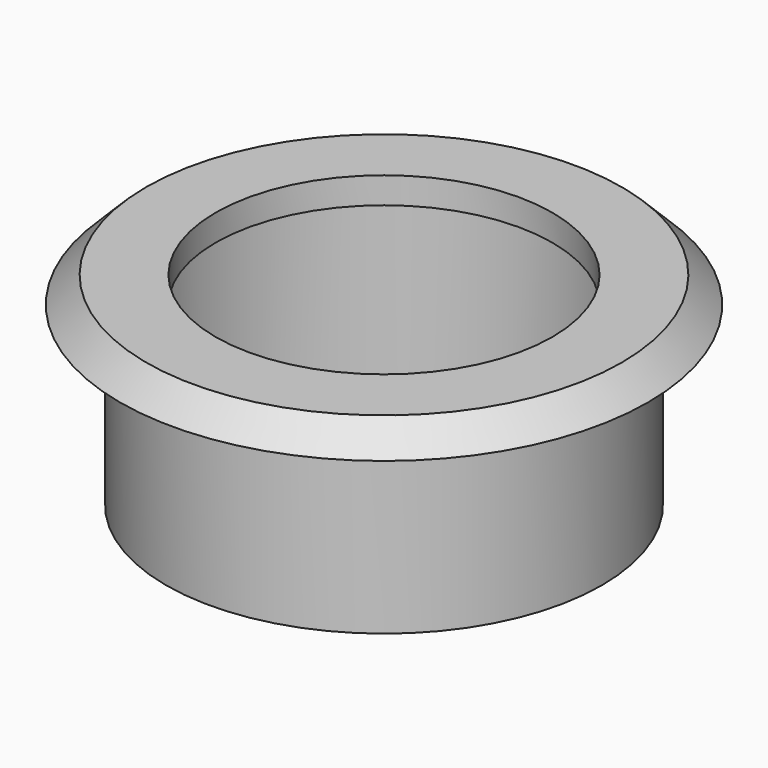
from build123d import *

# Parameters (mm, degrees)
F0_R     = 30
F1_DEPTH = 3
F2_SIZE  = 2.99999
F3_R     = 19.125
F4_DEPTH = 3.001
F5_R     = 24.75
F5_R_2   = 22.75
F6_DEPTH = 20


# Not quite as in the source:
# - a fillet or chamfer is up to 0.001 mm smaller than in the source, because OpenCascade refuses the exact size


with BuildPart() as f1:
    # F0 (on Top) → F1 (new body)
    with BuildSketch(Plane.XY):
        Circle(F0_R)
    extrude(amount=F1_DEPTH)

    # F2 (size 3 in the source; OpenCascade refuses exactly that, so slightly less here)
    f2_edges = [f1.edges().sort_by_distance(p)[0] for p in [
        (-30, 0, 3),
    ]]
    chamfer(f2_edges, length=F2_SIZE)

    # F3 (on face) → F4 (cut, through all)
    with BuildSketch(Plane.XY.offset(3)):
        Circle(F3_R)
    extrude(amount=-F4_DEPTH, mode=Mode.SUBTRACT)

    # F5 (on face) → F6 (join)
    with BuildSketch(Plane(origin=(0, 0, 0), x_dir=(1, 0, 0), z_dir=(0, 0, -1))):
        Circle(F5_R)
        Circle(F5_R_2, mode=Mode.SUBTRACT)
    extrude(amount=F6_DEPTH)


solid = f1.part
